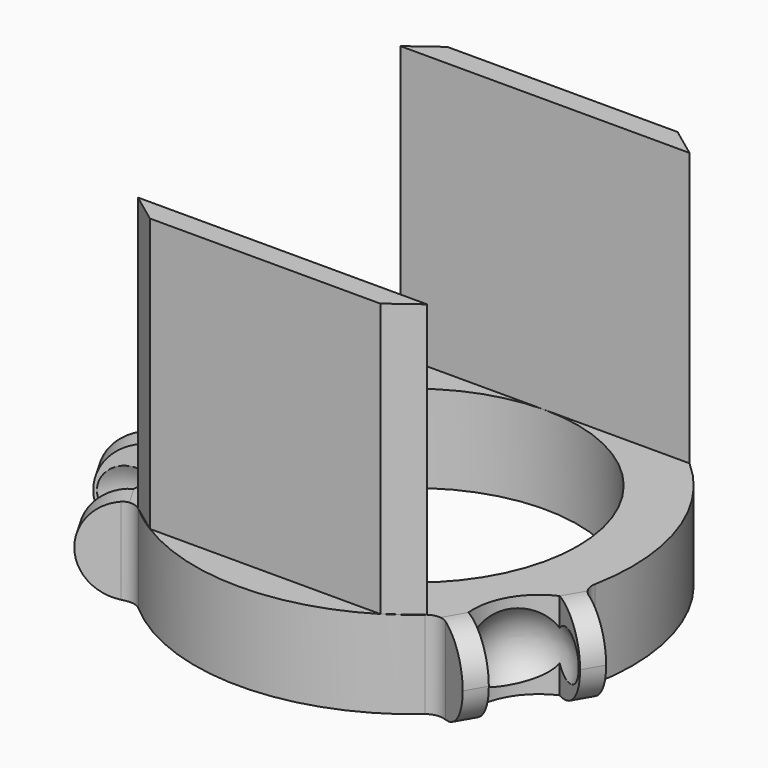
from build123d import *

# Parameters (mm, degrees)
F0_R            = 15
F2_DEPTH        = 8
F5_COPIES_COUNT = 3
F6_R            = 3.99999
F7_R            = 1.5
F9_DEPTH        = 25


# Not quite as in the source:
# - a fillet or chamfer is up to 0.001 mm smaller than in the source, because OpenCascade refuses the exact size
# - a pattern or mirror of a feature is missing from the dataset's text; its kind, count and spacing are read off the source's solid


with BuildPart() as f2:
    # F0 (on Top) → F2 (new body)
    with BuildSketch(Plane.XY):
        with BuildLine():
            Line((-5.5, 23.6913686675), (-5.5, 19.228884523))
            ThreePointArc((-5.5, 19.228884523), (-17.3205080757, 10), (-19.4027024834, -4.8513025407))
            Line((-19.4027024834, -4.8513025407), (-23.2673271165, -7.0825446129))
            Line((-23.2673271165, -7.0825446129), (-22.2673271165, -8.8145954205))
            Line((-22.2673271165, -8.8145954205), (-18.8032255014, -6.8145954205))
            ThreePointArc((-18.8032255014, -6.8145954205), (-16.0775588327, -9.28238292), (-15.3032255014, -12.876773247))
            Line((-15.3032255014, -12.876773247), (-18.7673271165, -14.876773247))
            Line((-18.7673271165, -14.876773247), (-17.7673271165, -16.6088240546))
            Line((-17.7673271165, -16.6088240546), (-13.9027024834, -14.3775819823))
            ThreePointArc((-13.9027024834, -14.3775819823), (0, -20), (13.9027024834, -14.3775819823))
            Line((13.9027024834, -14.3775819823), (17.7673271165, -16.6088240546))
            Line((17.7673271165, -16.6088240546), (18.7673271165, -14.876773247))
            Line((18.7673271165, -14.876773247), (15.3032255014, -12.876773247))
            ThreePointArc((15.3032255014, -12.876773247), (16.0775588327, -9.28238292), (18.8032255014, -6.8145954205))
            Line((18.8032255014, -6.8145954205), (22.2673271165, -8.8145954205))
            Line((22.2673271165, -8.8145954205), (23.2673271165, -7.0825446129))
            Line((23.2673271165, -7.0825446129), (19.4027024834, -4.8513025407))
            ThreePointArc((19.4027024834, -4.8513025407), (17.3205080757, 10), (5.5, 19.228884523))
            Line((5.5, 19.228884523), (5.5, 23.6913686675))
            Line((5.5, 23.6913686675), (3.5, 23.6913686675))
            Line((3.5, 23.6913686675), (3.5, 19.6913686675))
            ThreePointArc((3.5, 19.6913686675), (0, 18.5647658399), (-3.5, 19.6913686675))
            Line((-3.5, 19.6913686675), (-3.5, 23.6913686675))
            Line((-3.5, 23.6913686675), (-5.5, 23.6913686675))
        make_face()
        Circle(F0_R, mode=Mode.SUBTRACT)
    extrude(amount=F2_DEPTH)

    # F4 (on offset) → F5 (revolve, cut)
    with BuildSketch(Plane.XY.offset(4)):
        with BuildLine():
            Line((0, 17.1913686675), (0, 25.3913686675))
            ThreePointArc((0, 25.3913686675), (-4.1, 21.2913686675), (0, 17.1913686675))
        make_face()
    f5 = revolve(axis=Axis((0, 21.2913686675, 4), (0, -1, 0)), mode=Mode.SUBTRACT)

    # F5_copies: F5 ×3 about axis
    f5_copies_axis = Axis((0, 0, 0), (0, 0, 1))
    for i in range(1, F5_COPIES_COUNT):
        add(f5.rotate(f5_copies_axis, i * 360 / F5_COPIES_COUNT), mode=Mode.SUBTRACT)

    # F6 (radius 4 in the source; OpenCascade refuses exactly that, so slightly less here)
    f6_edges = [f2.edges().sort_by_distance(p)[0] for p in [
        (-4.5, 23.691369, 8),
        (4.5, 23.691369, 8),
        (22.767327, -7.94857, 8),
        (18.267327, -15.742799, 8),
        (-18.267327, -15.742799, 8),
        (-22.767327, -7.94857, 8),
        (-18.267327, -15.742799, 0),
        (-22.767327, -7.94857, 0),
        (18.267327, -15.742799, 0),
        (22.767327, -7.94857, 0),
        (4.5, 23.691369, 0),
        (-4.5, 23.691369, 0),
    ]]
    fillet(f6_edges, radius=F6_R)

    # F7
    f7_edges = [f2.edges().sort_by_distance(p)[0] for p in [
        (-19.402702, -4.851303, 4),
        (-5.5, 19.228885, 4),
        (5.5, 19.228885, 4),
        (19.402702, -4.851303, 4),
        (13.902702, -14.377582, 4),
        (-13.902702, -14.377582, 4),
    ]]
    fillet(f7_edges, radius=F7_R)

    # F8 (on face) → F9 (join)
    with BuildSketch(Plane.XY.offset(8)):
        Polygon((-10.5356537529, 17), (-13.2287565553, 15), (-1.63e-08, 15), (13.2287565553, 15), (10.5356537529, 17), align=None)
        Polygon((13.2287565553, -15), (0, -15), (-13.2287565553, -15), (-10.5356537529, -17), (10.5356537529, -17), align=None)
    extrude(amount=F9_DEPTH)


solid = f2.part
